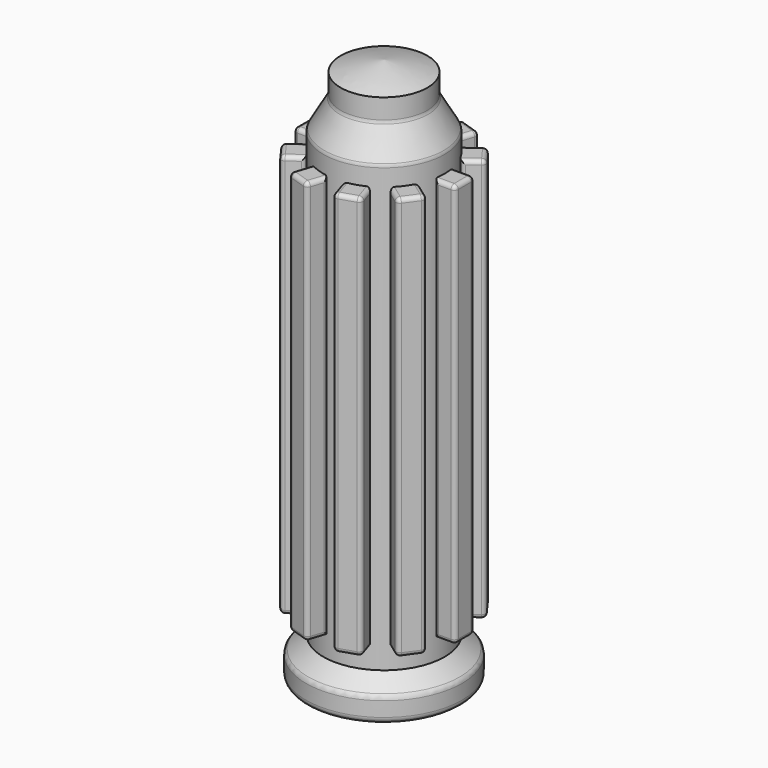
from build123d import *

# Parameters (mm, degrees)
F2_R     = 1.6
F4_W     = 6
F4_H     = 100
F6_R     = 1
F7_COUNT = 10


with BuildPart() as f1:
    # F0 (on Front) → F1 (revolve)
    with BuildSketch(Plane.XZ):
        with BuildLine():
            Line((10.75, 125), (10.75, 0))
            Line((10.75, 0), (19.325, 0))
            Line((19.325, 0), (19.325, 6))
            Line((19.325, 6), (15, 9.6291059048))
            Line((15, 9.6291059048), (15, 119.6291059048))
            Line((15, 119.6291059048), (10.74441231, 127))
            Line((10.74441231, 127), (10.74441231, 132.369821592))
            ThreePointArc((10.74441231, 132.369821592), (5.4257767556, 133.9037494188), (0, 135))
            Line((0, 135), (0, 125))
            Line((0, 125), (10.75, 125))
        make_face()
    revolve(axis=Axis((0, 0, 89.3560386384), (0, 0, 1)))

    # F2
    f2_edges = [f1.edges().sort_by_distance(p)[0] for p in [
        (-15, 0, 119.629106),
        (-10.744412, 0, 127),
        (12.872206, 0, 123.314553),
        (-19.325, 0, 0),
        (-19.325, 0, 6),
        (19.325, 0, 3),
    ]]
    fillet(f2_edges, radius=F2_R)


with BuildPart() as f5:
    # F4 (on offset) → F5 (new body, up to the next surface of F1)
    with BuildSketch(Plane.YZ.offset(20)):
        with Locations((0, 65)):
            Rectangle(F4_W, F4_H)
    extrude(until=Until.NEXT, target=f1.part, dir=(-1, 0, 0))

    # F6
    f6_edges = [f5.edges().sort_by_distance(p)[0] for p in [
        (20, -3, 65),
        (20, 3, 65),
        (14.696938, -3, 65),
        (14.696938, 3, 65),
        (20, 0, 115),
        (17.348469, 3, 115),
        (17.348469, -3, 115),
        (20, 0, 15),
        (17.348469, 3, 15),
        (17.348469, -3, 15),
    ]]
    fillet(f6_edges, radius=F6_R)


with BuildPart() as f7_1:
    # F7: instance of F5
    add(f5.part.rotate(Axis((0, 0, 9.6291059048), (0, 0, 1)), 1 * 360 / F7_COUNT))


with BuildPart() as f7_2:
    # F7: instance of F5
    add(f5.part.rotate(Axis((0, 0, 9.6291059048), (0, 0, 1)), 2 * 360 / F7_COUNT))


with BuildPart() as f7_3:
    # F7: instance of F5
    add(f5.part.rotate(Axis((0, 0, 9.6291059048), (0, 0, 1)), 3 * 360 / F7_COUNT))


with BuildPart() as f7_4:
    # F7: instance of F5
    add(f5.part.rotate(Axis((0, 0, 9.6291059048), (0, 0, 1)), 4 * 360 / F7_COUNT))


with BuildPart() as f7_5:
    # F7: instance of F5
    add(f5.part.rotate(Axis((0, 0, 9.6291059048), (0, 0, 1)), 5 * 360 / F7_COUNT))


with BuildPart() as f7_6:
    # F7: instance of F5
    add(f5.part.rotate(Axis((0, 0, 9.6291059048), (0, 0, 1)), 6 * 360 / F7_COUNT))


with BuildPart() as f7_7:
    # F7: instance of F5
    add(f5.part.rotate(Axis((0, 0, 9.6291059048), (0, 0, 1)), 7 * 360 / F7_COUNT))


with BuildPart() as f7_8:
    # F7: instance of F5
    add(f5.part.rotate(Axis((0, 0, 9.6291059048), (0, 0, 1)), 8 * 360 / F7_COUNT))


with BuildPart() as f7_9:
    # F7: instance of F5
    add(f5.part.rotate(Axis((0, 0, 9.6291059048), (0, 0, 1)), 9 * 360 / F7_COUNT))


solid = Compound([f1.part, f5.part, f7_1.part, f7_2.part, f7_3.part, f7_4.part, f7_5.part, f7_6.part, f7_7.part, f7_8.part, f7_9.part])
